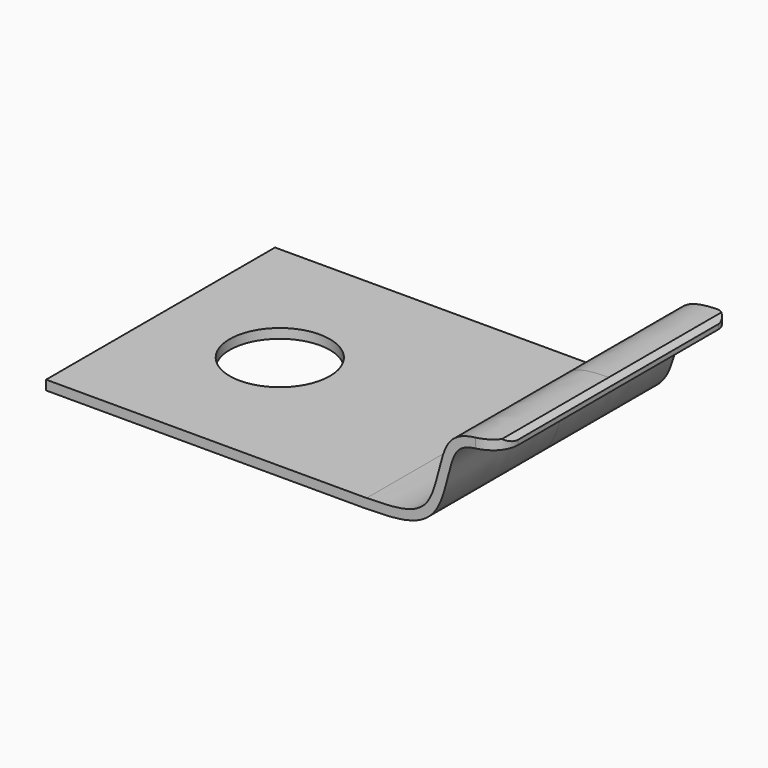
from build123d import *

# Parameters (mm, degrees)
F1_DEPTH    = 60
F2_R        = 21
F3_DEPTH    = 25.4
F4_T1_DEPTH = 65.200331563
F4_T3_DEPTH = 65.200331563
F5_R        = 10
F6_R        = 5


# Not quite as in the source:
# - a fillet or chamfer that OpenCascade refuses, or shapes differently, is made with other operations: its cross-section is extruded or revolved along the edge and cut away or added
# - the dataset's text gives a spline's control points without its knots; the knots are read off the source's solid


with BuildPart() as f1:
    # F0 (on Front) → F1 (new body, symmetric)
    with BuildSketch(Plane.XZ):
        with BuildLine():
            Line((0, 4), (0, 0))
            Line((0, 0), (134.4173699617, 0))
            Line((134.4173699617, 0), (134.5156762737, 0.0012081988))
            add(Edge.make_bspline(
                [(134.5156762737, 0.0012081988), (136.4412649676, 0.0485468782), (140.2763156439, 0.119434119), (145.8743978066, 0.4044797047), (150.3510695403, 1.0273190491), (153.7894078511, 1.9429841158), (156.2802330282, 2.8986647279), (158.2547462203, 3.9721610511), (159.742379044, 5.0235711097), (160.8019653259, 5.9125281204), (161.7935655068, 6.9010122474), (162.711452768, 7.9959327427), (163.5213429004, 9.1503598515), (164.4758269522, 10.7468127213), (165.4676861949, 12.8275263264), (166.42846639, 15.4079904943), (167.2304938066, 18.0312616598), (167.9298730275, 20.6536586802), (168.5732519985, 23.2263112252), (169.2005944517, 25.6940527379), (169.8453183168, 27.9950302112), (170.4178385402, 29.7159633299), (170.9015265062, 30.937033126), (171.2758440473, 31.7654748423), (171.5948760116, 32.3754073451), (171.8519779723, 32.8118865449), (172.1083616356, 33.2119555054), (172.4402204212, 33.6666398475), (172.9971831192, 34.3103142087), (173.7543203787, 34.9884401126), (174.8266057385, 35.6724492135), (176.1342158241, 36.2558320856), (177.7208250124, 36.7365981264), (180.2271678507, 37.2306981317), (184.0858279898, 37.5657574861), (187.8939372956, 37.5942963604), (189.9681193063, 37.5777642449)],
                knots=[0, 0, 0, 0, 0.0625, 0.125, 0.1875, 0.21875, 0.25, 0.28125, 0.296875, 0.3125, 0.328125, 0.34375, 0.359375, 0.375, 0.40625, 0.4375, 0.46875, 0.5, 0.53125, 0.5625, 0.59375, 0.625, 0.640625, 0.65625, 0.671875, 0.6796875, 0.6875, 0.703125, 0.71875, 0.75, 0.78125, 0.8125, 0.84375, 0.875, 0.9375, 1, 1, 1, 1], degree=3))
            Line((189.9681193063, 37.5777642449), (190, 41.5776371956))
            add(Edge.make_bspline(
                [(134.4173699617, 4), (144.934588281, 4.2585553329), (164.0700073734, 4.0486560983), (164.7009353827, 40.1911626223), (179.3143613789, 41.6628062936), (190, 41.5776371956)],
                knots=[0, 0, 0, 0, 0.3385935841, 0.6837265028, 1, 1, 1, 1], degree=3))
            Line((134.4173699617, 4), (0, 4))
        make_face()
    extrude(amount=F1_DEPTH, both=True)

    # F2 (on face) → F3 (cut)
    with BuildSketch(Plane.XY.offset(4)):
        with Locations((50, 0)):
            Circle(F2_R)
    extrude(amount=-F3_DEPTH, mode=Mode.SUBTRACT)

    # F4: chamfer of 2 on 2 edges, made by hand

    # F4_s2 → F4_t1 (cut)
    with BuildSketch(Plane.XZ.offset(-65.200331563)):
        with BuildLine():
            Line((190.0404149328, 39.5104765848), (187.920796438, 41.6398005777))
            Line((187.920796438, 41.6398005777), (187.9206603648, 41.6798003463))
            ThreePointArc((187.9206603648, 41.6798003463), (188.9604383984, 41.6233187105), (190.0003188069, 41.6176359251))
            Line((190.0003188069, 41.6176359251), (190.0399987295, 41.5773183887))
            ThreePointArc((190.0399987295, 41.5773183887), (190.0317624605, 40.5439647919), (190.0804136623, 39.5101577778))
            Line((190.0804136623, 39.5101577778), (190.0404149328, 39.5104765848))
        make_face()
    extrude(amount=F4_T1_DEPTH, mode=Mode.SUBTRACT)

    # F4_s4 → F4_t3 (cut)
    with BuildSketch(Plane.XZ):
        with BuildLine():
            Line((190.0404149328, 39.5104765848), (187.920796438, 41.6398005777))
            Line((187.920796438, 41.6398005777), (187.9206603648, 41.6798003463))
            ThreePointArc((187.9206603648, 41.6798003463), (188.9604383984, 41.6233187105), (190.0003188069, 41.6176359251))
            Line((190.0003188069, 41.6176359251), (190.0399987295, 41.5773183887))
            ThreePointArc((190.0399987295, 41.5773183887), (190.0317624605, 40.5439647919), (190.0804136623, 39.5101577778))
            Line((190.0804136623, 39.5101577778), (190.0404149328, 39.5104765848))
        make_face()
    extrude(amount=F4_T3_DEPTH, mode=Mode.SUBTRACT)

    # F5
    f5_edges = [f1.edges().sort_by_distance(p)[0] for p in [
        (189.976048, -60, 38.572469),
    ]]
    fillet(f5_edges, radius=F5_R)

    # F6
    f6_edges = [f1.edges().sort_by_distance(p)[0] for p in [
        (189.976048, 60, 38.572469),
    ]]
    fillet(f6_edges, radius=F6_R)


solid = f1.part
